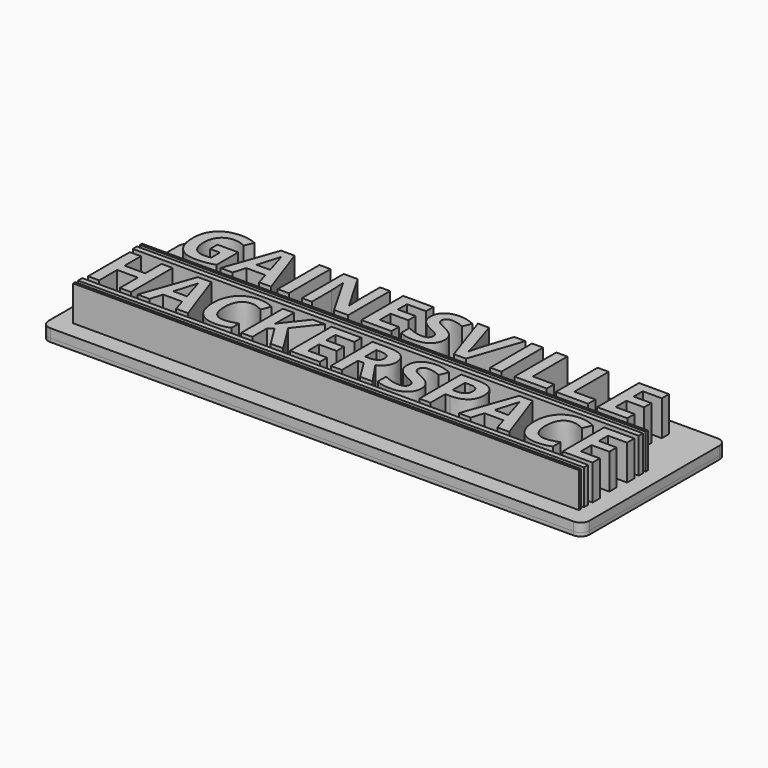
from build123d import *

# Parameters (mm, degrees)
F3_DEPTH     = 5
F4_DEPTH     = 2
F0_TEXT_SIZE = 41.6666666667
F5_DEPTH     = 25
F1_W         = 288
F1_H         = 3
F1_H_2       = 1.5
F6_DEPTH     = 25


# Not quite as in the source:
# - Text() gives the source's letters only with a copy of the font that has no kerning and outlines rounded to 1/6400 em; it was checked with that copy


with BuildPart() as f3:
    # F2 (on Top) → F3 (new body)
    with BuildSketch(Plane.XY):
        with BuildLine():
            Line((149, 40), (-149, 40))
            ThreePointArc((-149, 40), (-152.5355339059, 38.5355339059), (-154, 35))
            Line((-154, 35), (-154, -57.5))
            ThreePointArc((-154, -57.5), (-152.5355339059, -61.0355339059), (-149, -62.5))
            Line((-149, -62.5), (149, -62.5))
            ThreePointArc((149, -62.5), (152.5355339059, -61.0355339059), (154, -57.5))
            Line((154, -57.5), (154, 35))
            ThreePointArc((154, 35), (152.5355339059, 38.5355339059), (149, 40))
        make_face()
    extrude(amount=F3_DEPTH)


with BuildPart() as f4:
    # F4 (new): a face of the model
    f4_faces = [f3.part.faces().sort_by_distance(p)[0] for p in [
        (0, -11.25, 0),
    ]]
    extrude(f4_faces, amount=F4_DEPTH)

    # F0 (on Top) → F5 (join)
    with BuildSketch(Plane.XY):
        with Locations((-132.2005208333, 0)):
            Text('GAINESVILLE', F0_TEXT_SIZE, font='Open Sans', font_style=FontStyle.BOLD, text_align=(TextAlign.LEFT, TextAlign.BOTTOM))
        with Locations((-146.8391927083, -43)):
            Text('HACKERSPACE', F0_TEXT_SIZE, font='Open Sans', font_style=FontStyle.BOLD, text_align=(TextAlign.LEFT, TextAlign.BOTTOM))
    extrude(amount=F5_DEPTH)

    # F1 (on Top) → F6 (join)
    with BuildSketch(Plane.XY):
        with Locations((0, -8.5)):
            Rectangle(F1_W, F1_H)
        with Locations((0, -4.25)):
            Rectangle(F1_W, F1_H_2)
        with Locations((0, -47.5)):
            Rectangle(F1_W, F1_H)
        with Locations((0, -51.75)):
            Rectangle(F1_W, F1_H_2)
    extrude(amount=F6_DEPTH)


solid = Compound([f3.part, f4.part])
